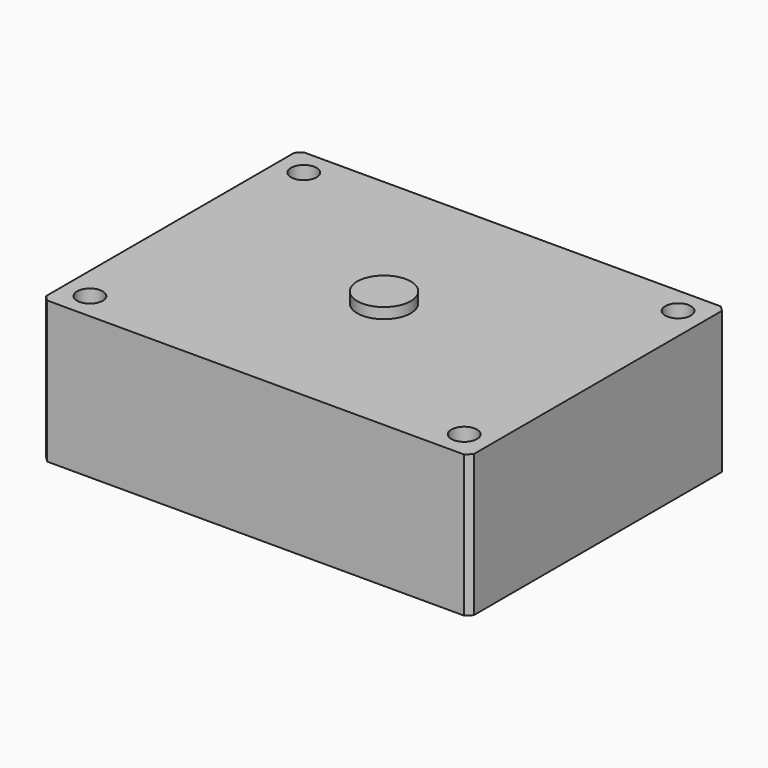
from build123d import *

# Parameters (mm, degrees)
F0_W      = 4000
F0_H      = 3000
F1_DEPTH  = 100
F2_SIZE   = 50
F4_D      = 200
F5_R      = 120
F5_R_2    = 100
F6_DEPTH  = 50
F7_DEPTH  = 1126.6541127115
F9_R      = 250
F10_DEPTH = 100


with BuildPart() as f1:
    # F0 (on Top) → F1 (new body, symmetric)
    with BuildSketch(Plane.XY):
        Rectangle(F0_W, F0_H)
    extrude(amount=F1_DEPTH, both=True)

    # F2
    f2_edges = [f1.edges().sort_by_distance(p)[0] for p in [
        (-2000, -1500, 0),
        (2000, 1500, 0),
        (2000, -1500, 0),
        (-2000, 1500, 0),
    ]]
    chamfer(f2_edges, length=F2_SIZE)

    # F4 (through all)
    with Locations(Plane.XY.offset(100)):
        with Locations((-1750, 1250), (1750, 1250), (-1750, -1250), (1750, -1250)):
            Hole(F4_D / 2)

    # F5 (on face) → F6 (cut)
    with BuildSketch(Plane.XY.offset(100)):
        with Locations((-1750, -1250)):
            Circle(F5_R)
        with Locations((-1750, -1250)):
            Circle(F5_R_2, mode=Mode.SUBTRACT)
        with Locations((-1750, 1250)):
            Circle(F5_R)
        with Locations((-1750, 1250)):
            Circle(F5_R_2, mode=Mode.SUBTRACT)
        with Locations((1750, 1250)):
            Circle(F5_R)
        with Locations((1750, 1250)):
            Circle(F5_R_2, mode=Mode.SUBTRACT)
        with Locations((1750, -1250)):
            Circle(F5_R)
        with Locations((1750, -1250)):
            Circle(F5_R_2, mode=Mode.SUBTRACT)
    extrude(amount=-F6_DEPTH, mode=Mode.SUBTRACT)

    # F7 (add): a face of the model
    f7_faces = [f1.faces().sort_by_distance(p)[0] for p in [
        (0, 0, 100),
    ]]
    extrude(f7_faces, amount=F7_DEPTH)


with BuildPart() as f10:
    # F9 (on face) → F10 (new body)
    with BuildSketch(Plane.XY.offset(1226.6541127115)):
        Circle(F9_R)
    extrude(amount=F10_DEPTH)


solid = Compound([f1.part, f10.part])
